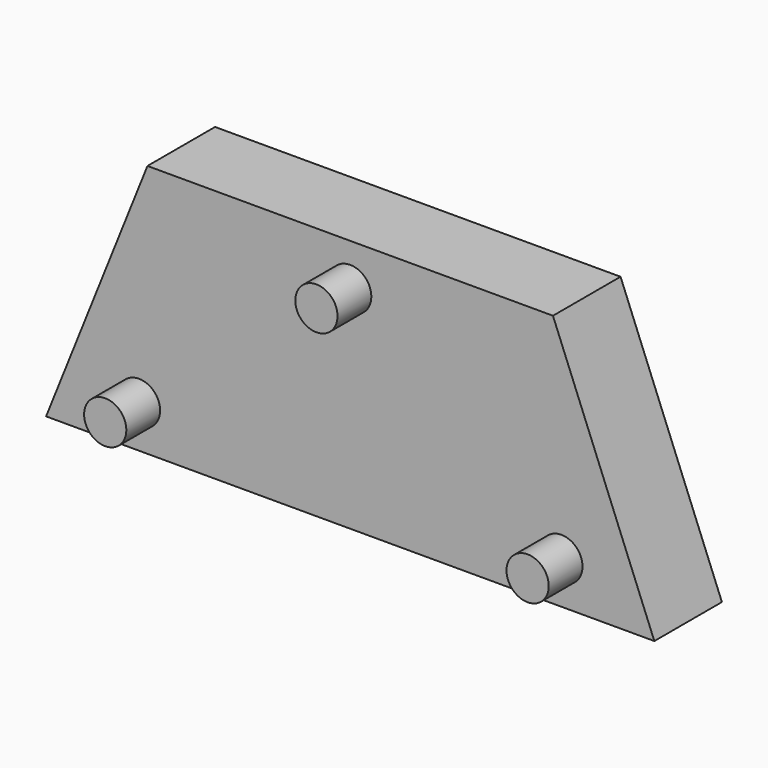
from build123d import *

# Parameters (mm, degrees)
F1_DEPTH = 6.35
F2_R     = 1.5875
F3_DEPTH = 3.175


# Not quite as in the source:
# - a feature of the source that left no trace in its solid (it failed there, or was rolled back) is left out


with BuildPart() as f1:
    # F0 (on Front) → F1 (new body)
    with BuildSketch(Plane.XZ):
        Polygon((-57.817878572, 25.3623127937), (-65.437878572, 6.3123127937), (-19.717878572, 6.3123127937), (-27.337878572, 25.3623127937), (-42.577878572, 25.3623127937), align=None)
    extrude(amount=F1_DEPTH)

    # F2 (on face) → F3 (join)
    with BuildSketch(Plane.XZ.offset(6.35)):
        with Locations((-58.452878572, 9.4873127937)):
            Circle(F2_R)
        with Locations((-26.702878572, 9.4873127937)):
            Circle(F2_R)
        with Locations((-42.577878572, 22.1873127937)):
            Circle(F2_R)
    extrude(amount=F3_DEPTH)


solid = f1.part
